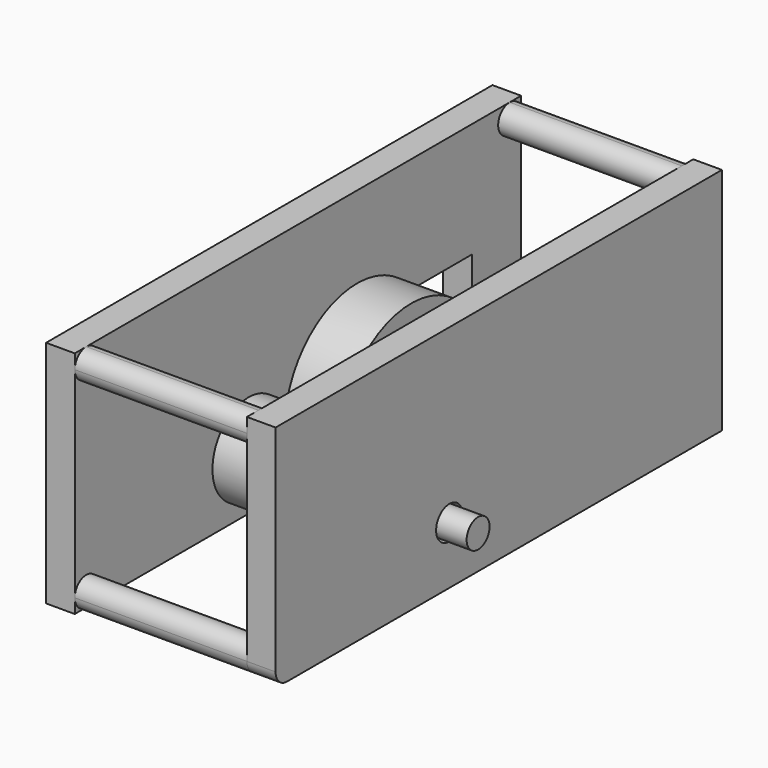
from build123d import *

# Parameters (mm, degrees)
F0_R      = 5
F0_R_2    = 1.8415
F0_R_3    = 1.5875
F1_DEPTH  = 3.175
F2_DEPTH  = 19.05
F3_R      = 1.8415
F4_DEPTH  = 3.175
F3_R_2    = 1.5875
F5_DEPTH  = 3.175
F6_DEPTH  = 6
F7_DEPTH  = 6
F8_DEPTH  = 3.175
F9_DEPTH  = 25.4
F10_DEPTH = 6


# Not quite as in the source:
# - a feature names something its author has since deleted; it is built from what else it names


with BuildPart() as f1:
    # F0 (on Right) → F1 (new body)
    with BuildSketch(Plane.YZ):
        with BuildLine():
            ThreePointArc((18.4078367749, 6.35), (25.0352423421, 15.7641174197), (36.1329581332, 12.7))
            Line((36.1329581332, 12.7), (44.2828367749, 12.7))
            Line((44.2828367749, 12.7), (44.2828367749, 0))
            Line((44.2828367749, 0), (49.5203367749, 0))
            ThreePointArc((49.5203367749, 0), (48.3978047598, 2.7100320151), (51.1078367749, 1.5875))
            Line((51.1078367749, 1.5875), (51.1078367749, 23.8125))
            ThreePointArc((51.1078367749, 23.8125), (48.3978047598, 22.6899679849), (49.5203367749, 25.4))
            Line((49.5203367749, 25.4), (41.8216693056, 25.4))
            Line((41.8216693056, 25.4), (35.8211970083, 25.4))
            Line((35.8211970083, 25.4), (-9.0546632251, 25.4))
            ThreePointArc((-9.0546632251, 25.4), (-7.9321312099, 24.9350320151), (-7.4671632251, 23.8125))
            ThreePointArc((-7.4671632251, 23.8125), (-9.0546632251, 22.225), (-10.6421632251, 23.8125))
            Line((-10.6421632251, 23.8125), (-10.6421632251, 1.5875))
            ThreePointArc((-10.6421632251, 1.5875), (-9.0546632251, 3.175), (-7.4671632251, 1.5875))
            ThreePointArc((-7.4671632251, 1.5875), (-7.9321312099, 0.4649679849), (-9.0546632251, 0))
            Line((-9.0546632251, 0), (20.6827154167, 0))
            ThreePointArc((20.6827154167, 0), (18.9937193553, 2.9774055671), (18.4078367749, 6.35))
        make_face()
        with Locations((13.4078367749, 6.35)):
            Circle(F0_R, mode=Mode.SUBTRACT)
        with BuildLine():
            ThreePointArc((36.1329581332, 0), (37.8219541946, 2.9774055671), (38.4078367749, 6.35))
            ThreePointArc((38.4078367749, 6.35), (37.8219541946, 9.7225944329), (36.1329581332, 12.7))
            Line((36.1329581332, 12.7), (22.0578367749, 12.7))
            Line((22.0578367749, 12.7), (22.0578367749, 0))
            Line((22.0578367749, 0), (36.1329581332, 0))
        make_face()
        with Locations((28.4078367749, 6.35)):
            Circle(F0_R_2, mode=Mode.SUBTRACT)
        with BuildLine():
            ThreePointArc((36.1329581332, 12.7), (37.8219541946, 9.7225944329), (38.4078367749, 6.35))
            ThreePointArc((38.4078367749, 6.35), (37.8219541946, 2.9774055671), (36.1329581332, 0))
            Line((36.1329581332, 0), (43.4878367749, 0))
            Line((43.4878367749, 0), (44.2828367749, 0))
            Line((44.2828367749, 0), (44.2828367749, 12.7))
            Line((44.2828367749, 12.7), (36.1329581332, 12.7))
        make_face()
        with Locations((13.4078367749, 6.35)):
            Circle(F0_R)
        with Locations((13.4078367749, 6.35)):
            Circle(F0_R_2, mode=Mode.SUBTRACT)
        with BuildLine():
            Line((22.0578367749, 12.7), (36.1329581332, 12.7))
            ThreePointArc((36.1329581332, 12.7), (25.0352423421, 15.7641174197), (18.4078367749, 6.35))
            ThreePointArc((18.4078367749, 6.35), (18.9937193553, 2.9774055671), (20.6827154167, 0))
            Line((20.6827154167, 0), (22.0578367749, 0))
            Line((22.0578367749, 0), (22.0578367749, 12.7))
        make_face()
        with Locations((28.4078367749, 6.35)):
            Circle(F0_R_2)
        with Locations((28.4078367749, 6.35)):
            Circle(F0_R_3, mode=Mode.SUBTRACT)
        with BuildLine():
            ThreePointArc((-10.6421632251, 1.5875), (-10.1771952402, 0.4649679849), (-9.0546632251, 0))
            ThreePointArc((-9.0546632251, 0), (-7.9321312099, 0.4649679849), (-7.4671632251, 1.5875))
            ThreePointArc((-7.4671632251, 1.5875), (-9.0546632251, 3.175), (-10.6421632251, 1.5875))
        make_face()
        with BuildLine():
            ThreePointArc((51.1078367749, 1.5875), (48.3978047598, 2.7100320151), (49.5203367749, 0))
            ThreePointArc((49.5203367749, 0), (50.6428687901, 0.4649679849), (51.1078367749, 1.5875))
        make_face()
        with BuildLine():
            ThreePointArc((-9.0546632251, 25.4), (-10.1771952402, 24.9350320151), (-10.6421632251, 23.8125))
            ThreePointArc((-10.6421632251, 23.8125), (-9.0546632251, 22.225), (-7.4671632251, 23.8125))
            ThreePointArc((-7.4671632251, 23.8125), (-7.9321312099, 24.9350320151), (-9.0546632251, 25.4))
        make_face()
        with BuildLine():
            ThreePointArc((49.5203367749, 25.4), (48.3978047598, 22.6899679849), (51.1078367749, 23.8125))
            ThreePointArc((51.1078367749, 23.8125), (50.6428687901, 24.9350320151), (49.5203367749, 25.4))
        make_face()
        with Locations((28.4078367749, 6.35)):
            Circle(F0_R_3)
        with BuildLine():
            ThreePointArc((51.1078367749, 1.5875), (50.6428687901, 0.4649679849), (49.5203367749, 0))
            Line((49.5203367749, 0), (50.2833090723, 0))
            Line((50.2833090723, 0), (51.1078367749, 0))
            Line((51.1078367749, 0), (51.1078367749, 1.5875))
        make_face()
        with BuildLine():
            Line((-10.6421632251, 25.4), (-10.6421632251, 23.8125))
            ThreePointArc((-10.6421632251, 23.8125), (-10.1771952402, 24.9350320151), (-9.0546632251, 25.4))
            Line((-9.0546632251, 25.4), (-10.6421632251, 25.4))
        make_face()
        with BuildLine():
            ThreePointArc((49.5203367749, 25.4), (50.6428687901, 24.9350320151), (51.1078367749, 23.8125))
            Line((51.1078367749, 23.8125), (51.1078367749, 25.4))
            Line((51.1078367749, 25.4), (49.5203367749, 25.4))
        make_face()
    extrude(amount=F1_DEPTH)


with BuildPart() as f2:
    # F0 (on Right) → F2 (new body)
    with BuildSketch(Plane.YZ):
        with BuildLine():
            ThreePointArc((-10.6421632251, 1.5875), (-10.1771952402, 0.4649679849), (-9.0546632251, 0))
            ThreePointArc((-9.0546632251, 0), (-7.9321312099, 0.4649679849), (-7.4671632251, 1.5875))
            ThreePointArc((-7.4671632251, 1.5875), (-9.0546632251, 3.175), (-10.6421632251, 1.5875))
        make_face()
    extrude(amount=-F2_DEPTH)


with BuildPart() as f2b:
    # F0 (on Right) → F2, piece 2 (new body)
    with BuildSketch(Plane.YZ):
        with BuildLine():
            ThreePointArc((51.1078367749, 1.5875), (48.3978047598, 2.7100320151), (49.5203367749, 0))
            ThreePointArc((49.5203367749, 0), (50.6428687901, 0.4649679849), (51.1078367749, 1.5875))
        make_face()
    extrude(amount=-F2_DEPTH)


with BuildPart() as f2c:
    # F0 (on Right) → F2, piece 3 (new body)
    with BuildSketch(Plane.YZ):
        with BuildLine():
            ThreePointArc((-9.0546632251, 25.4), (-10.1771952402, 24.9350320151), (-10.6421632251, 23.8125))
            ThreePointArc((-10.6421632251, 23.8125), (-9.0546632251, 22.225), (-7.4671632251, 23.8125))
            ThreePointArc((-7.4671632251, 23.8125), (-7.9321312099, 24.9350320151), (-9.0546632251, 25.4))
        make_face()
    extrude(amount=-F2_DEPTH)


with BuildPart() as f2d:
    # F0 (on Right) → F2, piece 4 (new body)
    with BuildSketch(Plane.YZ):
        with BuildLine():
            ThreePointArc((49.5203367749, 25.4), (48.3978047598, 22.6899679849), (51.1078367749, 23.8125))
            ThreePointArc((51.1078367749, 23.8125), (50.6428687901, 24.9350320151), (49.5203367749, 25.4))
        make_face()
    extrude(amount=-F2_DEPTH)


with BuildPart() as f4:
    # F3 (on face) → F4 (new body)
    with BuildSketch(Plane(origin=(-19.05, 0, 0), x_dir=(0, -1, 0), z_dir=(-1, 0, 0))):
        with BuildLine():
            Line((10.6421632251, 25.4), (-49.5203367749, 25.4))
            ThreePointArc((-49.5203367749, 25.4), (-48.3978047598, 24.9350320151), (-47.9328367749, 23.8125))
            ThreePointArc((-47.9328367749, 23.8125), (-49.5203367749, 22.225), (-51.1078367749, 23.8125))
            Line((-51.1078367749, 23.8125), (-51.1078367749, 0))
            Line((-51.1078367749, 0), (-44.2828367749, 0))
            Line((-44.2828367749, 0), (-44.2828367749, 12.7))
            Line((-44.2828367749, 12.7), (-36.1329581332, 12.7))
            ThreePointArc((-36.1329581332, 12.7), (-25.0352423421, 15.7641174197), (-18.4078367749, 6.35))
            ThreePointArc((-18.4078367749, 6.35), (-18.9937193553, 2.9774055671), (-20.6827154167, 0))
            Line((-20.6827154167, 0), (10.6421632251, 0))
            Line((10.6421632251, 0), (10.6421632251, 25.4))
        make_face()
        with BuildLine():
            ThreePointArc((-8.4078367749, 6.35), (-13.4078367749, 1.35), (-18.4078367749, 6.35))
            ThreePointArc((-18.4078367749, 6.35), (-13.4078367749, 11.35), (-8.4078367749, 6.35))
        make_face(mode=Mode.SUBTRACT)
        with BuildLine():
            ThreePointArc((-8.4078367749, 6.35), (-13.4078367749, 11.35), (-18.4078367749, 6.35))
            ThreePointArc((-18.4078367749, 6.35), (-13.4078367749, 1.35), (-8.4078367749, 6.35))
        make_face()
        with Locations((-13.4078367749, 6.35)):
            Circle(F3_R, mode=Mode.SUBTRACT)
        with BuildLine():
            Line((-22.0578367749, 0), (-20.6827154167, 0))
            ThreePointArc((-20.6827154167, 0), (-18.9937193553, 2.9774055671), (-18.4078367749, 6.35))
            ThreePointArc((-18.4078367749, 6.35), (-25.0352423421, 15.7641174197), (-36.1329581332, 12.7))
            Line((-36.1329581332, 12.7), (-22.0578367749, 12.7))
            Line((-22.0578367749, 12.7), (-22.0578367749, 6.35))
            Line((-22.0578367749, 6.35), (-22.0578367749, 0))
        make_face()
        with BuildLine():
            ThreePointArc((-47.9328367749, 23.8125), (-48.3978047598, 24.9350320151), (-49.5203367749, 25.4))
            ThreePointArc((-49.5203367749, 25.4), (-50.6428687901, 24.9350320151), (-51.1078367749, 23.8125))
            ThreePointArc((-51.1078367749, 23.8125), (-49.5203367749, 22.225), (-47.9328367749, 23.8125))
        make_face()
        with BuildLine():
            Line((-49.5203367749, 25.4), (-51.1078367749, 25.4))
            Line((-51.1078367749, 25.4), (-51.1078367749, 23.8125))
            ThreePointArc((-51.1078367749, 23.8125), (-50.6428687901, 24.9350320151), (-49.5203367749, 25.4))
        make_face()
    extrude(amount=F4_DEPTH)


with BuildPart() as f5:
    # F3 (on face) → F5 (new body)
    with BuildSketch(Plane(origin=(-19.05, 0, 0), x_dir=(0, -1, 0), z_dir=(-1, 0, 0))):
        with Locations((-28.4078367749, 6.35)):
            Circle(F3_R_2)
    extrude(amount=F5_DEPTH)

    # F3 (on face) → F6 (join)
    with BuildSketch(Plane(origin=(-19.05, 0, 0), x_dir=(0, -1, 0), z_dir=(-1, 0, 0))):
        with Locations((-28.4078367749, 6.35)):
            Circle(F3_R_2)
    extrude(amount=-F6_DEPTH)


with BuildPart() as f7:
    # F3 (on face) → F7 (new body)
    with BuildSketch(Plane(origin=(-19.05, 0, 0), x_dir=(0, -1, 0), z_dir=(-1, 0, 0))):
        with BuildLine():
            ThreePointArc((-36.1329581332, 12.7), (-38.4078367749, 6.35), (-36.1329581332, 0))
            Line((-36.1329581332, 0), (-22.0578367749, 0))
            Line((-22.0578367749, 0), (-22.0578367749, 6.35))
            Line((-22.0578367749, 6.35), (-22.0578367749, 12.7))
            Line((-22.0578367749, 12.7), (-36.1329581332, 12.7))
        make_face()
        with Locations((-28.4078367749, 6.35)):
            Circle(F3_R, mode=Mode.SUBTRACT)
        with BuildLine():
            Line((-22.0578367749, 0), (-20.6827154167, 0))
            ThreePointArc((-20.6827154167, 0), (-18.9937193553, 2.9774055671), (-18.4078367749, 6.35))
            ThreePointArc((-18.4078367749, 6.35), (-25.0352423421, 15.7641174197), (-36.1329581332, 12.7))
            Line((-36.1329581332, 12.7), (-22.0578367749, 12.7))
            Line((-22.0578367749, 12.7), (-22.0578367749, 6.35))
            Line((-22.0578367749, 6.35), (-22.0578367749, 0))
        make_face()
        with BuildLine():
            ThreePointArc((-36.1329581332, 0), (-28.4078367749, -3.65), (-20.6827154167, 0))
            Line((-20.6827154167, 0), (-22.0578367749, 0))
            Line((-22.0578367749, 0), (-36.1329581332, 0))
        make_face()
        with Locations((-28.4078367749, 6.35)):
            Circle(F3_R)
        with Locations((-28.4078367749, 6.35)):
            Circle(F3_R_2, mode=Mode.SUBTRACT)
    extrude(amount=-F7_DEPTH)


with BuildPart() as f8:
    # F3 (on face) → F8 (new body)
    with BuildSketch(Plane(origin=(-19.05, 0, 0), x_dir=(0, -1, 0), z_dir=(-1, 0, 0))):
        with Locations((-13.4078367749, 6.35)):
            Circle(F3_R_2)
    extrude(amount=F8_DEPTH)

    # F3 (on face) → F9 (join)
    with BuildSketch(Plane(origin=(-19.05, 0, 0), x_dir=(0, -1, 0), z_dir=(-1, 0, 0))):
        with Locations((-13.4078367749, 6.35)):
            Circle(F3_R_2)
    extrude(amount=-F9_DEPTH)


with BuildPart() as f10:
    # F3 (on face) → F10 (new body)
    with BuildSketch(Plane(origin=(-19.05, 0, 0), x_dir=(0, -1, 0), z_dir=(-1, 0, 0))):
        with BuildLine():
            ThreePointArc((-8.4078367749, 6.35), (-13.4078367749, 11.35), (-18.4078367749, 6.35))
            ThreePointArc((-18.4078367749, 6.35), (-13.4078367749, 1.35), (-8.4078367749, 6.35))
        make_face()
        with Locations((-13.4078367749, 6.35)):
            Circle(F3_R, mode=Mode.SUBTRACT)
        with Locations((-13.4078367749, 6.35)):
            Circle(F3_R)
        with Locations((-13.4078367749, 6.35)):
            Circle(F3_R_2, mode=Mode.SUBTRACT)
    extrude(amount=-F10_DEPTH)


solid = Compound([f1.part, f2.part, f2b.part, f2c.part, f2d.part, f4.part, f5.part, f7.part, f8.part, f10.part])
